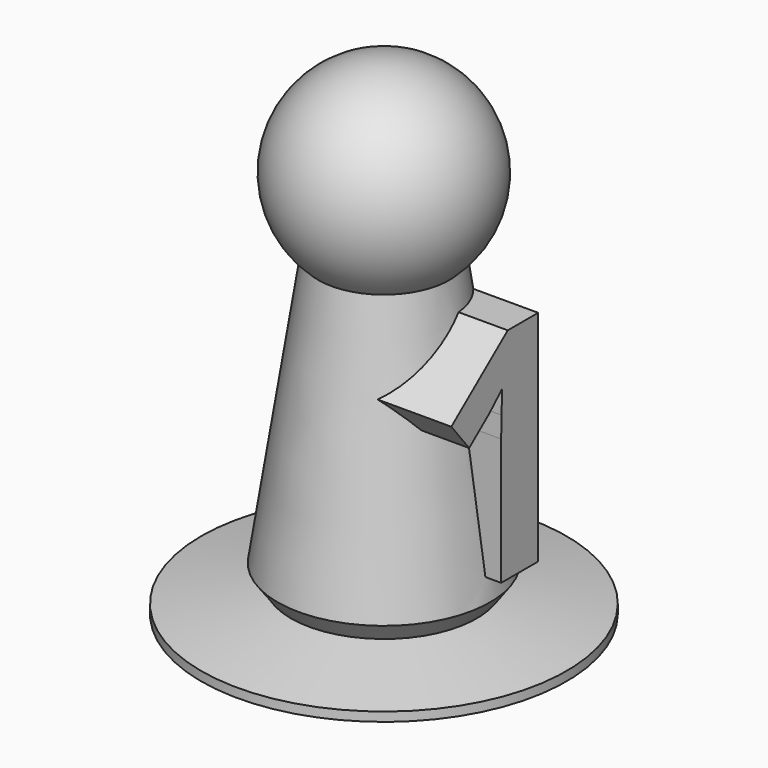
from build123d import *

# Parameters (mm, degrees)
F2_T         = -2.54
F3_TEXT_SIZE = 85.2921372926
F4_DEPTH     = 33.02


# Not quite as in the source:
# - Text() gives the source's letters only with a copy of the font that has no kerning and outlines rounded to 1/6400 em; it was checked with that copy


with BuildPart() as f1:
    # F0 (on Front) → F1 (revolve)
    with BuildSketch(Plane.XZ):
        with BuildLine():
            Line((-50.8, -75.0875837376), (0, -75.0875837376))
            Line((0, -75.0875837376), (0, 60.4993418939))
            ThreePointArc((0, 60.4993418939), (-25.6489479602, 42.7959642288), (-18.1925435981, 12.5357569227))
            Line((-18.1925435981, 12.5357569227), (-29.5651562948, -62.6245576696))
            Line((-29.5651562948, -62.6245576696), (-25.8522276922, -67.7759323592))
            Line((-25.8522276922, -67.7759323592), (-50.8, -72.5475837376))
            Line((-50.8, -72.5475837376), (-50.8, -75.0875837376))
        make_face()
    revolve(axis=Axis((0, 0, -7.2941209218), (0, 0, -1)))

    # F2
    f2_openings = [f1.faces().sort_by_distance(p)[0] for p in [
        (0, 0, -75.087584),
    ]]
    offset(amount=F2_T, openings=f2_openings, kind=Kind.INTERSECTION)

    # F3 (on Right) → F4 (join)
    with BuildSketch(Plane.YZ):
        with Locations((-22.8700488806, -56.5398631152)):
            Text('1', F3_TEXT_SIZE, font='Open Sans', font_style=FontStyle.BOLD, text_align=(TextAlign.LEFT, TextAlign.BOTTOM))
    extrude(amount=F4_DEPTH)


solid = f1.part
